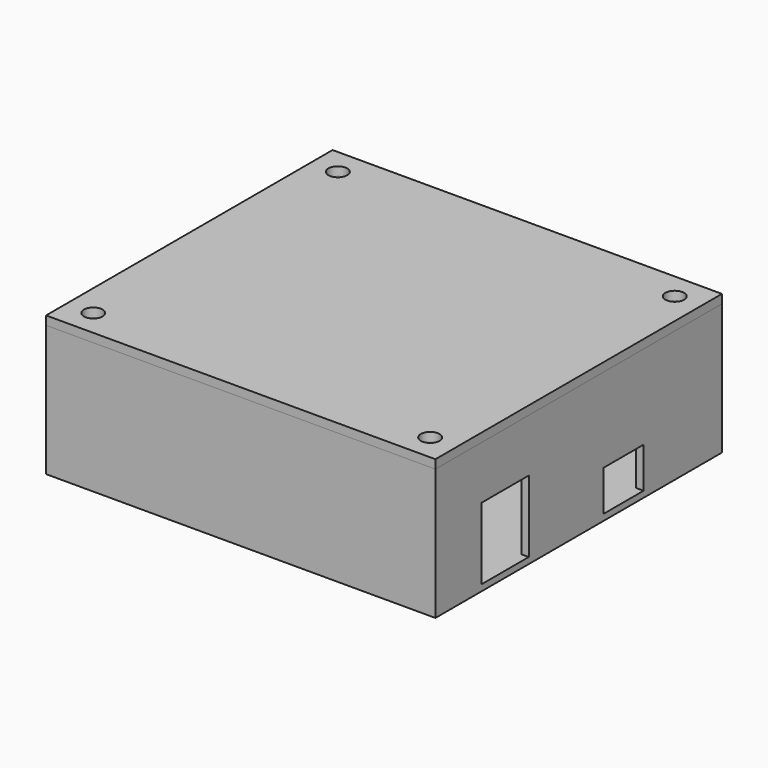
from build123d import *

# Parameters (mm, degrees)
F0_W     = 62.4
F0_H     = 57.4
F0_W_2   = 6
F0_H_2   = 6
F0_R     = 1.5
F1_DEPTH = 20
F2_W     = 62.4
F2_H     = 57.4
F3_DEPTH = 1
F4_W     = 9.5
F4_H     = 11.5
F4_W_2   = 8
F4_H_2   = 6.5
F5_DEPTH = 1.2
F7_DEPTH = 0.6
F6_W     = 62.4
F6_H     = 57.4
F6_R     = 1.5
F8_DEPTH = 1.4


with BuildPart() as f1:
    # F0 (on Top) → F1 (new body)
    with BuildSketch(Plane.XY):
        with Locations((0, -5)):
            Rectangle(F0_W, F0_H)
        Polygon((-30, 16.5), (-30, 22.5), (-24, 22.5), (24, 22.5), (30, 22.5), (30, 16.5), (30, -26.5), (30, -32.5), (24, -32.5), (-24, -32.5), (-30, -32.5), (-30, -26.5), align=None, mode=Mode.SUBTRACT)
        with Locations((27, -29.5)):
            Rectangle(F0_W_2, F0_H_2)
        with Locations((27, -29.5)):
            Circle(F0_R, mode=Mode.SUBTRACT)
        with Locations((-27, 19.5)):
            Rectangle(F0_W_2, F0_H_2)
        with Locations((-27, 19.5)):
            Circle(F0_R, mode=Mode.SUBTRACT)
        with Locations((-27, -29.5)):
            Rectangle(F0_W_2, F0_H_2)
        with Locations((-27, -29.5)):
            Circle(F0_R, mode=Mode.SUBTRACT)
        with Locations((27, 19.5)):
            Rectangle(F0_W_2, F0_H_2)
        with Locations((27, 19.5)):
            Circle(F0_R, mode=Mode.SUBTRACT)
    extrude(amount=F1_DEPTH)

    # F2 (on Top) → F3 (join)
    with BuildSketch(Plane.XY):
        with Locations((0, -5)):
            Rectangle(F2_W, F2_H)
    extrude(amount=-F3_DEPTH)

    # F4 (on face) → F5 (cut, through all)
    with BuildSketch(Plane.YZ.offset(31.2)):
        with Locations((-19.75, 5.75)):
            Rectangle(F4_W, F4_H)
        with Locations((4, 3.25)):
            Rectangle(F4_W_2, F4_H_2)
    extrude(amount=-F5_DEPTH, mode=Mode.SUBTRACT)


with BuildPart() as f7:
    # F6 (on face) → F7 (new body)
    with BuildSketch(Plane.XY.offset(20)):
        Polygon((24, 22.5), (-24, 22.5), (-24, 16.5), (-30, 16.5), (-30, -26.5), (-24, -26.5), (-24, -32.5), (24, -32.5), (24, -26.5), (30, -26.5), (30, 16.5), (24, 16.5), align=None)
    extrude(amount=-F7_DEPTH)

    # F6 (on face) → F8 (join)
    with BuildSketch(Plane.XY.offset(20)):
        with Locations((0, -5)):
            Rectangle(F6_W, F6_H)
        with Locations((-27, -29.5)):
            Circle(F6_R, mode=Mode.SUBTRACT)
        with Locations((27, -29.5)):
            Circle(F6_R, mode=Mode.SUBTRACT)
        with Locations((-27, 19.5)):
            Circle(F6_R, mode=Mode.SUBTRACT)
        Polygon((-24, 16.5), (-24, 22.5), (24, 22.5), (24, 16.5), (30, 16.5), (30, -26.5), (24, -26.5), (24, -32.5), (-24, -32.5), (-24, -26.5), (-30, -26.5), (-30, 16.5), align=None, mode=Mode.SUBTRACT)
        with Locations((27, 19.5)):
            Circle(F6_R, mode=Mode.SUBTRACT)
        Polygon((24, 22.5), (-24, 22.5), (-24, 16.5), (-30, 16.5), (-30, -26.5), (-24, -26.5), (-24, -32.5), (24, -32.5), (24, -26.5), (30, -26.5), (30, 16.5), (24, 16.5), align=None)
    extrude(amount=F8_DEPTH)


solid = Compound([f1.part, f7.part])
